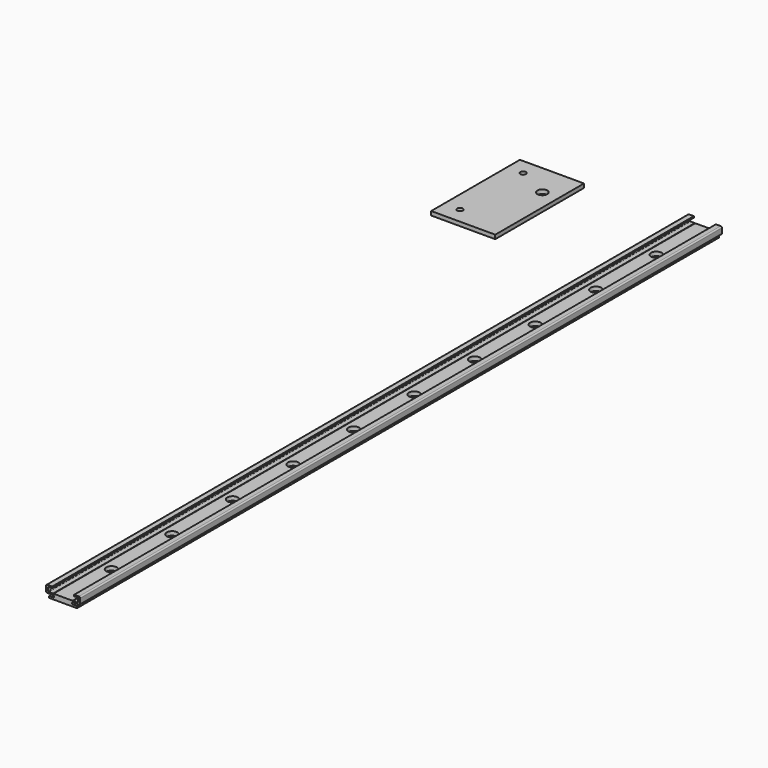
from build123d import *

# Parameters (mm, degrees)
F1_DEPTH = 636
F2_R     = 2.25
F3_DEPTH = 4.101
F2_R_2   = 4.25
F4_DEPTH = 3.0988
F5_W     = 50.8
F5_H     = 87.939999888
F5_R     = 2.25
F5_R_2   = 3.96875
F6_DEPTH = 3.175


# Not quite as in the source:
# - a feature names something its author has since deleted; it is built from what else it names


with BuildPart() as f1:
    # F0 (on Front) → F1 (new body)
    with BuildSketch(Plane.XZ):
        with BuildLine():
            Line((22.9752515742, 4.1), (19.4252515742, 4.1))
            ThreePointArc((19.4252515742, 4.1), (19.0716981836, 4.2464466094), (18.9252515742, 4.6))
            Line((18.9252515742, 4.6), (18.9252515742, 7.1))
            ThreePointArc((18.9252515742, 7.1), (19.0716981836, 7.4535533906), (19.4252515742, 7.6))
            Line((19.4252515742, 7.6), (22.1752515742, 7.6))
            Line((22.1752515742, 7.6), (22.1752515742, 8.7))
            Line((22.1752515742, 8.7), (18.6321558738, 8.7))
            ThreePointArc((18.6321558738, 8.7), (17.7936560083, 8.4836800987), (17.4252515742, 7.7))
            Line((17.4252515742, 7.7), (17.4252515742, 4))
            ThreePointArc((17.4252515742, 4), (17.718144793, 3.2928932188), (18.4252515742, 3))
            Line((18.4252515742, 3), (23.1252515742, 3))
            ThreePointArc((23.1252515742, 3), (23.8752515742, 2.25), (23.1252515742, 1.5))
            Line((23.1252515742, 1.5), (20.1252515742, 1.5))
            ThreePointArc((20.1252515742, 1.5), (19.983830218, 1.4414213562), (19.9252515742, 1.3))
            Line((19.9252515742, 1.3), (19.9252515742, 0))
            Line((19.9252515742, 0), (41.9252515742, 0))
            Line((41.9252515742, 0), (41.9252515742, 1.3))
            ThreePointArc((41.9252515742, 1.3), (41.8666729304, 1.4414213562), (41.7252515742, 1.5))
            Line((41.7252515742, 1.5), (38.7252515742, 1.5))
            ThreePointArc((38.7252515742, 1.5), (37.9752515742, 2.25), (38.7252515742, 3))
            Line((38.7252515742, 3), (38.9860151642, 3))
            Line((38.9860151642, 3), (43.4252515742, 3))
            ThreePointArc((43.4252515742, 3), (44.1323583554, 3.2928932188), (44.4252515742, 4))
            Line((44.4252515742, 4), (44.4252515742, 7.7))
            ThreePointArc((44.4252515742, 7.7), (44.1323583554, 8.4071067812), (43.4252515742, 8.7))
            Line((43.4252515742, 8.7), (39.6752515742, 8.7))
            Line((39.6752515742, 8.7), (39.6752515742, 7.6))
            Line((39.6752515742, 7.6), (42.4252515742, 7.6))
            ThreePointArc((42.4252515742, 7.6), (42.7788049648, 7.4535533906), (42.9252515742, 7.1))
            Line((42.9252515742, 7.1), (42.9252515742, 4.6))
            ThreePointArc((42.9252515742, 4.6), (42.7788049648, 4.2464466094), (42.4252515742, 4.1))
            Line((42.4252515742, 4.1), (38.8752515742, 4.1))
            ThreePointArc((38.8752515742, 4.1), (38.6752515742, 3.8913035005), (38.4752515742, 4.1))
            Line((38.4752515742, 4.1), (23.3752515742, 4.1))
            ThreePointArc((23.3752515742, 4.1), (23.1752515742, 3.9086639286), (22.9752515742, 4.1))
        make_face()
    extrude(amount=F1_DEPTH)

    # F2 (on face) → F3 (cut, through all)
    with BuildSketch(Plane.XY.offset(4.1)):
        with Locations((30.9252515742, -48)):
            Circle(F2_R)
        with Locations((30.9252515742, -108)):
            Circle(F2_R)
        with Locations((30.9252515742, -168)):
            Circle(F2_R)
        with Locations((30.9252515742, -228)):
            Circle(F2_R)
        with Locations((30.9252515742, -288)):
            Circle(F2_R)
        with Locations((30.9252515742, -348)):
            Circle(F2_R)
        with Locations((30.9252515742, -408)):
            Circle(F2_R)
        with Locations((30.9252515742, -468)):
            Circle(F2_R)
        with Locations((30.9252515742, -528)):
            Circle(F2_R)
        with Locations((30.9252515742, -588)):
            Circle(F2_R)
    extrude(amount=-F3_DEPTH, mode=Mode.SUBTRACT)

    # F2 (on face) → F4 (cut)
    with BuildSketch(Plane.XY.offset(4.1)):
        with Locations((30.9252515742, -108)):
            Circle(F2_R_2)
        with Locations((30.9252515742, -108)):
            Circle(F2_R, mode=Mode.SUBTRACT)
        with Locations((30.9252515742, -48)):
            Circle(F2_R_2)
        with Locations((30.9252515742, -48)):
            Circle(F2_R, mode=Mode.SUBTRACT)
        with Locations((30.9252515742, -168)):
            Circle(F2_R_2)
        with Locations((30.9252515742, -168)):
            Circle(F2_R, mode=Mode.SUBTRACT)
        with Locations((30.9252515742, -228)):
            Circle(F2_R_2)
        with Locations((30.9252515742, -228)):
            Circle(F2_R, mode=Mode.SUBTRACT)
        with Locations((30.9252515742, -288)):
            Circle(F2_R_2)
        with Locations((30.9252515742, -288)):
            Circle(F2_R, mode=Mode.SUBTRACT)
        with Locations((30.9252515742, -348)):
            Circle(F2_R_2)
        with Locations((30.9252515742, -348)):
            Circle(F2_R, mode=Mode.SUBTRACT)
        with Locations((30.9252515742, -408)):
            Circle(F2_R_2)
        with Locations((30.9252515742, -408)):
            Circle(F2_R, mode=Mode.SUBTRACT)
        with Locations((30.9252515742, -468)):
            Circle(F2_R_2)
        with Locations((30.9252515742, -468)):
            Circle(F2_R, mode=Mode.SUBTRACT)
        with Locations((30.9252515742, -528)):
            Circle(F2_R_2)
        with Locations((30.9252515742, -528)):
            Circle(F2_R, mode=Mode.SUBTRACT)
        with Locations((30.9252515742, -588)):
            Circle(F2_R_2)
        with Locations((30.9252515742, -588)):
            Circle(F2_R, mode=Mode.SUBTRACT)
    extrude(amount=-F4_DEPTH, mode=Mode.SUBTRACT)


with BuildPart() as f6:
    # F5 (on Top) → F6 (new body)
    with BuildSketch(Plane.XY):
        with Locations((-90.3261050073, -43.969999944)):
            Rectangle(F5_W, F5_H)
        with Locations((-103.0261050073, -75.239999888)):
            Circle(F5_R, mode=Mode.SUBTRACT)
        with Locations((-103.0261050073, -12.7)):
            Circle(F5_R, mode=Mode.SUBTRACT)
        with Locations((-77.6261050073, -25.4)):
            Circle(F5_R_2, mode=Mode.SUBTRACT)
    extrude(amount=F6_DEPTH)


solid = Compound([f1.part, f6.part])
